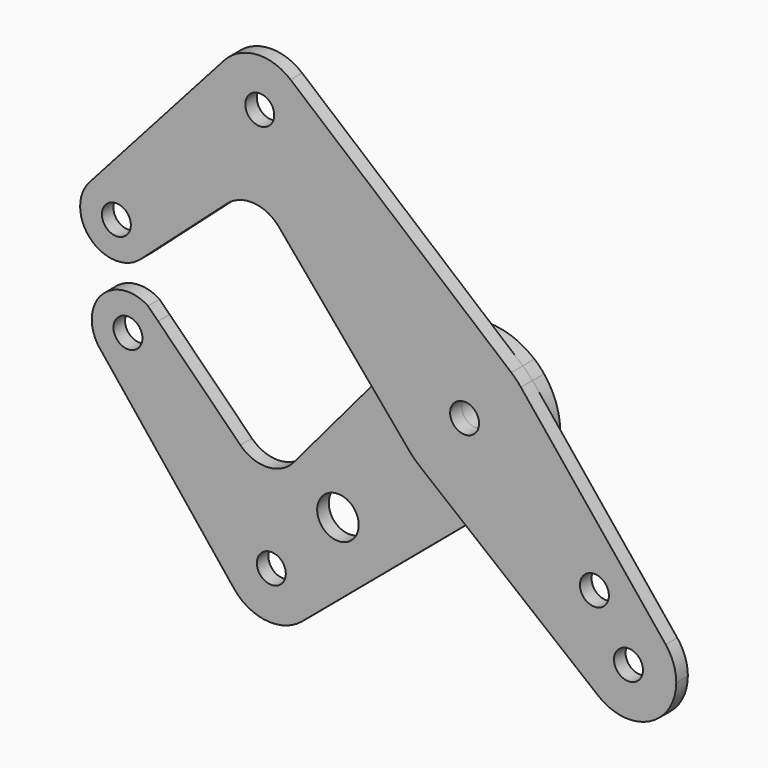
from build123d import *

# Parameters (mm, degrees)
F0_R     = 3.175
F0_R_2   = 3.9751
F1_DEPTH = 3.175
F0_R_3   = 4.55279125
F2_DEPTH = 3.175


# Not quite as in the source:
# - a feature names something its author has since deleted; it is built from what else it names


with BuildPart() as f1:
    # F0 (on Front) → F1 (new body)
    with BuildSketch(Plane.XZ):
        with BuildLine():
            ThreePointArc((-82.2563895183, 18.7531498051), (-73.5054766898, 20.8875043398), (-68.3946770291, 13.4703841816))
            ThreePointArc((-68.3946770291, 13.4703841816), (-69.08870209, 10.2244671992), (-71.0494114056, 7.5461716924))
            Line((-71.0494114056, 7.5461716924), (-52.0712687873, 24.4694470818))
            ThreePointArc((-52.0712687873, 24.4694470818), (-46.2149635715, 26.465847689), (-40.7009159693, 23.6592117657))
            Line((-40.7009159693, 23.6592117657), (-20.7610835727, 0))
            Line((-20.7610835727, 0), (-12.1388473833, 10.2305429575))
            ThreePointArc((-12.1388473833, 10.2305429575), (-1.349375, 15.817547601), (10.2305429575, 12.1388473833))
            Line((10.2305429575, 12.1388473833), (-38.1491222534, 52.9129198783))
            ThreePointArc((-38.1491222534, 52.9129198783), (-35.4006557474, 49.3189874266), (-34.4237806053, 44.9012806053))
            ThreePointArc((-34.4237806053, 44.9012806053), (-48.6325250533, 35.1106819965), (-52.7212410911, 51.8745312283))
            Line((-52.7212410911, 51.8745312283), (-82.2563895183, 18.7531498051))
        make_face()
        with BuildLine():
            ThreePointArc((-71.0494114056, 7.5461716924), (-69.08870209, 10.2244671992), (-68.3946770291, 13.4703841816))
            ThreePointArc((-68.3946770291, 13.4703841816), (-73.5054766898, 20.8875043398), (-82.2563895183, 18.7531498051))
            ThreePointArc((-82.2563895183, 18.7531498051), (-81.9448371048, 7.8577241059), (-71.0494114056, 7.5461716924))
        make_face()
        with Locations((-76.3321770291, 13.4703841816)):
            Circle(F0_R, mode=Mode.SUBTRACT)
        with BuildLine():
            ThreePointArc((-38.1491222534, 52.9129198783), (-45.6460041086, 55.35228023), (-52.7212410911, 51.8745312283))
            ThreePointArc((-52.7212410911, 51.8745312283), (-48.6325250533, 35.1106819965), (-34.4237806053, 44.9012806053))
            ThreePointArc((-34.4237806053, 44.9012806053), (-35.4006557474, 49.3189874266), (-38.1491222534, 52.9129198783))
        make_face()
        with Locations((-44.9012806053, 44.9012806053)):
            Circle(F0_R, mode=Mode.SUBTRACT)
        with BuildLine():
            Line((-12.1388473833, 10.2305429575), (-20.7610835727, 0))
            Line((-20.7610835727, 0), (-12.1388473833, -10.2305429575))
            ThreePointArc((-12.1388473833, -10.2305429575), (-15.875, 0), (-12.1388473833, 10.2305429575))
        make_face()
        with BuildLine():
            ThreePointArc((10.2305429575, -12.1388473833), (0.1694484732, -15.8740956346), (-9.9690883749, -12.354468907))
            Line((-9.9690883749, -12.354468907), (0.2196387976, -20.5759733985))
            Line((0.2196387976, -20.5759733985), (10.2305429575, -12.1388473833))
        make_face()
        with BuildLine():
            Line((44.0749739629, -29.3414261569), (12.354468907, 9.9690883749))
            ThreePointArc((12.354468907, 9.9690883749), (14.9690149793, 5.2862288591), (15.875, 0))
            ThreePointArc((15.875, 0), (14.3948861484, -6.6934951837), (10.2305429575, -12.1388473833))
            Line((10.2305429575, -12.1388473833), (0.2196387976, -20.5759733985))
            Line((0.2196387976, -20.5759733985), (29.3414261569, -44.0749739629))
            ThreePointArc((29.3414261569, -44.0749739629), (28.5123131844, -28.5123131844), (44.0749739629, -29.3414261569))
        make_face()
        with Locations((28.4592052015, -23.969077141)):
            Circle(F0_R, mode=Mode.SUBTRACT)
        with BuildLine():
            ThreePointArc((46.3985244843, -35.9210244843), (45.8005743706, -32.4321134373), (44.0749739629, -29.3414261569))
            ThreePointArc((44.0749739629, -29.3414261569), (28.5123131844, -28.5123131844), (29.3414261569, -44.0749739629))
            ThreePointArc((29.3414261569, -44.0749739629), (40.4398885437, -45.3739538642), (46.3985244843, -35.9210244843))
        make_face()
        with Locations((35.9210244843, -35.9210244843)):
            Circle(F0_R, mode=Mode.SUBTRACT)
        with BuildLine():
            ThreePointArc((12.354468907, 9.9690883749), (11.3444988329, 11.1048625039), (10.2305429575, 12.1388473833))
            ThreePointArc((10.2305429575, 12.1388473833), (-1.349375, 15.817547601), (-12.1388473833, 10.2305429575))
            ThreePointArc((-12.1388473833, 10.2305429575), (-15.875, 0), (-12.1388473833, -10.2305429575))
            ThreePointArc((-12.1388473833, -10.2305429575), (-11.1048625039, -11.3444988329), (-9.9690883749, -12.354468907))
            ThreePointArc((-9.9690883749, -12.354468907), (0.1694484732, -15.8740956346), (10.2305429575, -12.1388473833))
            ThreePointArc((10.2305429575, -12.1388473833), (14.3948861484, -6.6934951837), (15.875, 0))
            ThreePointArc((15.875, 0), (14.9690149793, 5.2862288591), (12.354468907, 9.9690883749))
        make_face()
        Circle(F0_R_2, mode=Mode.SUBTRACT)
        Circle(F0_R_2)
        Circle(F0_R, mode=Mode.SUBTRACT)
    extrude(amount=F1_DEPTH)


with BuildPart() as f2:
    # F0 (on Front) → F2 (new body)
    with BuildSketch(Plane.XZ):
        with BuildLine():
            Line((-12.1388473833, -10.2305429575), (-20.7610835727, 0))
            Line((-20.7610835727, 0), (-39.9810774323, -22.8051016586))
            ThreePointArc((-39.9810774323, -22.8051016586), (-45.7220225821, -25.6246494482), (-51.6818525337, -23.3032860773))
            Line((-51.6818525337, -23.3032860773), (-69.715236479, -5.2699021319))
            ThreePointArc((-69.715236479, -5.2699021319), (-68.7319838781, -7.3646480711), (-68.3946770291, -9.6539646322))
            ThreePointArc((-68.3946770291, -9.6539646322), (-73.7060338073, -17.144443791), (-82.5319439339, -14.6104549809))
            Line((-82.5319439339, -14.6104549809), (-53.0849729197, -51.4438478655))
            ThreePointArc((-53.0849729197, -51.4438478655), (-48.3677896582, -35.0138481157), (-34.4237806053, -44.9012806053))
            ThreePointArc((-34.4237806053, -44.9012806053), (-35.4006557474, -49.3189874266), (-38.1491222534, -52.9129198783))
            Line((-38.1491222534, -52.9129198783), (0.2196387976, -20.5759733985))
            Line((0.2196387976, -20.5759733985), (-9.9690883749, -12.354468907))
            ThreePointArc((-9.9690883749, -12.354468907), (-11.1048625039, -11.3444988329), (-12.1388473833, -10.2305429575))
        make_face()
        with Locations((-30.2993841525, -30.2993841525)):
            Circle(F0_R_3, mode=Mode.SUBTRACT)
        with BuildLine():
            ThreePointArc((12.354468907, 9.9690883749), (11.3444988329, 11.1048625039), (10.2305429575, 12.1388473833))
            ThreePointArc((10.2305429575, 12.1388473833), (-1.349375, 15.817547601), (-12.1388473833, 10.2305429575))
            ThreePointArc((-12.1388473833, 10.2305429575), (-15.875, 0), (-12.1388473833, -10.2305429575))
            ThreePointArc((-12.1388473833, -10.2305429575), (-11.1048625039, -11.3444988329), (-9.9690883749, -12.354468907))
            ThreePointArc((-9.9690883749, -12.354468907), (0.1694484732, -15.8740956346), (10.2305429575, -12.1388473833))
            ThreePointArc((10.2305429575, -12.1388473833), (14.3948861484, -6.6934951837), (15.875, 0))
            ThreePointArc((15.875, 0), (14.9690149793, 5.2862288591), (12.354468907, 9.9690883749))
        make_face()
        Circle(F0_R_2, mode=Mode.SUBTRACT)
        with BuildLine():
            ThreePointArc((-53.0849729197, -51.4438478655), (-45.9268855566, -55.3284633857), (-38.1491222534, -52.9129198783))
            ThreePointArc((-38.1491222534, -52.9129198783), (-35.4006557474, -49.3189874266), (-34.4237806053, -44.9012806053))
            ThreePointArc((-34.4237806053, -44.9012806053), (-48.3677896582, -35.0138481157), (-53.0849729197, -51.4438478655))
        make_face()
        with Locations((-44.9012806053, -44.9012806053)):
            Circle(F0_R, mode=Mode.SUBTRACT)
        with BuildLine():
            ThreePointArc((-68.3946770291, -9.6539646322), (-68.7319838781, -7.3646480711), (-69.715236479, -5.2699021319))
            Line((-69.715236479, -5.2699021319), (-71.9481145287, -3.0370240822))
            ThreePointArc((-71.9481145287, -3.0370240822), (-82.1896740468, -4.2973206328), (-82.5319439339, -14.6104549809))
            ThreePointArc((-82.5319439339, -14.6104549809), (-73.7060338073, -17.144443791), (-68.3946770291, -9.6539646322))
        make_face()
        with Locations((-76.3321770291, -9.6539646322)):
            Circle(F0_R, mode=Mode.SUBTRACT)
        Circle(F0_R_2)
        Circle(F0_R, mode=Mode.SUBTRACT)
        with BuildLine():
            Line((-12.1388473833, 10.2305429575), (-20.7610835727, 0))
            Line((-20.7610835727, 0), (-12.1388473833, -10.2305429575))
            ThreePointArc((-12.1388473833, -10.2305429575), (-15.875, 0), (-12.1388473833, 10.2305429575))
        make_face()
        with BuildLine():
            ThreePointArc((10.2305429575, -12.1388473833), (0.1694484732, -15.8740956346), (-9.9690883749, -12.354468907))
            Line((-9.9690883749, -12.354468907), (0.2196387976, -20.5759733985))
            Line((0.2196387976, -20.5759733985), (10.2305429575, -12.1388473833))
        make_face()
    extrude(amount=-F2_DEPTH)


solid = Compound([f1.part, f2.part])
